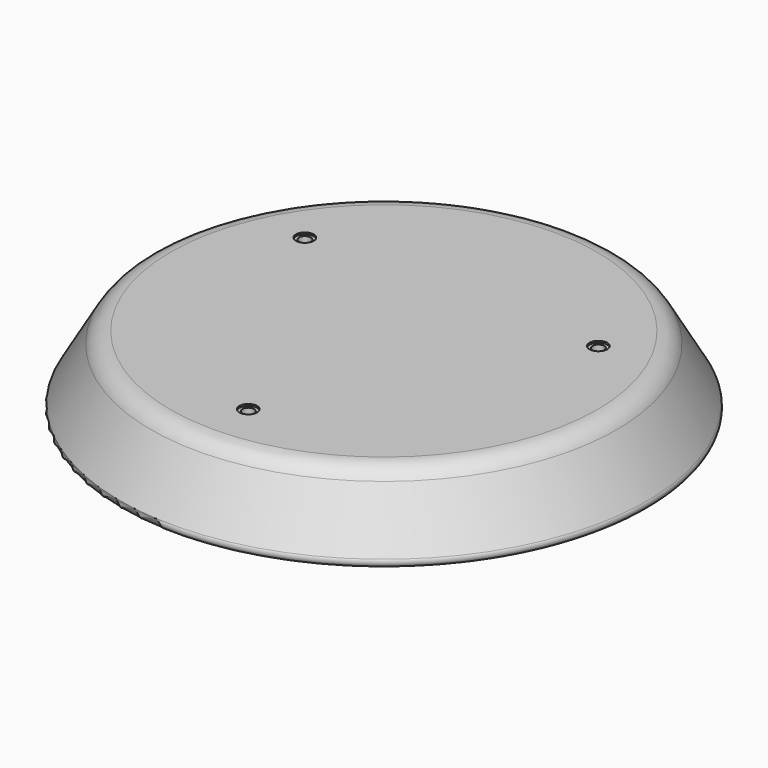
from build123d import *

# Parameters (mm, degrees)
F2_R     = 2.25
F2_R_2   = 1.65
F3_DEPTH = 10
F4_R     = 1.65
F5_DEPTH = 3
F6_R     = 2.5
F7_DEPTH = 0.5


# Not quite as in the source:
# - ends of sketch curves that miss each other by under 0.0002 mm in the source are joined


with BuildPart() as f1:
    # F0 (on Front) → F1 (revolve)
    with BuildSketch(Plane.XZ):
        with BuildLine():
            Line((0, 15.0000001043), (0, 18))
            Line((0, 18), (-60, 18))
            ThreePointArc((-60, 18), (-63.175, 17.149261314), (-65.499261314, 14.825))
            Line((-65.499261314, 14.825), (-74.0584790548, 0))
            ThreePointArc((-74.0584790548, 0), (-73.5094409491, -2.0490381057), (-71.4604028434, -1.5))
            Line((-71.4604028434, -1.5), (-62.901185193, 13.3250000522))
            ThreePointArc((-62.901185193, 13.3250000522), (-61.6750000522, 14.551185193), (-60, 15.0000001043))
            Line((-60, 15.0000001043), (0, 15.0000001043))
        make_face()
    revolve(axis=Axis((0, 0, 16.5000000522), (0, 0, -1)))

    # F2 (on face) → F3 (join)
    with BuildSketch(Plane(origin=(0, 0, 15.0000001043), x_dir=(1, 0, 0), z_dir=(0, 0, -1))):
        with Locations((0, 47.6650122409)):
            Circle(F2_R)
        with Locations((0, 47.6650122409)):
            Circle(F2_R_2, mode=Mode.SUBTRACT)
        with Locations((-41.2791114723, -23.8325061204)):
            Circle(F2_R)
        with Locations((-41.2791114723, -23.8325061204)):
            Circle(F2_R_2, mode=Mode.SUBTRACT)
        with Locations((41.2791114723, -23.8325061204)):
            Circle(F2_R)
        with Locations((41.2791114723, -23.8325061204)):
            Circle(F2_R_2, mode=Mode.SUBTRACT)
    extrude(amount=F3_DEPTH)

    # F4 (on face) → F5 (cut)
    with BuildSketch(Plane(origin=(0, 0, 15.0000001043), x_dir=(1, 0, 0), z_dir=(0, 0, -1))):
        with Locations((0, 47.6650122409)):
            Circle(F4_R)
        with Locations((-41.2791114723, -23.8325061204)):
            Circle(F4_R)
        with Locations((41.2791114723, -23.8325061204)):
            Circle(F4_R)
    extrude(amount=-F5_DEPTH, mode=Mode.SUBTRACT)

    # F6 (on face) → F7 (cut)
    with BuildSketch(Plane.XY.offset(18)):
        with Locations((0, -47.6650122409)):
            Circle(F6_R)
        with Locations((41.2791114723, 23.8325061204)):
            Circle(F6_R)
        with Locations((-41.2791114723, 23.8325061204)):
            Circle(F6_R)
    extrude(amount=-F7_DEPTH, mode=Mode.SUBTRACT)


solid = f1.part
